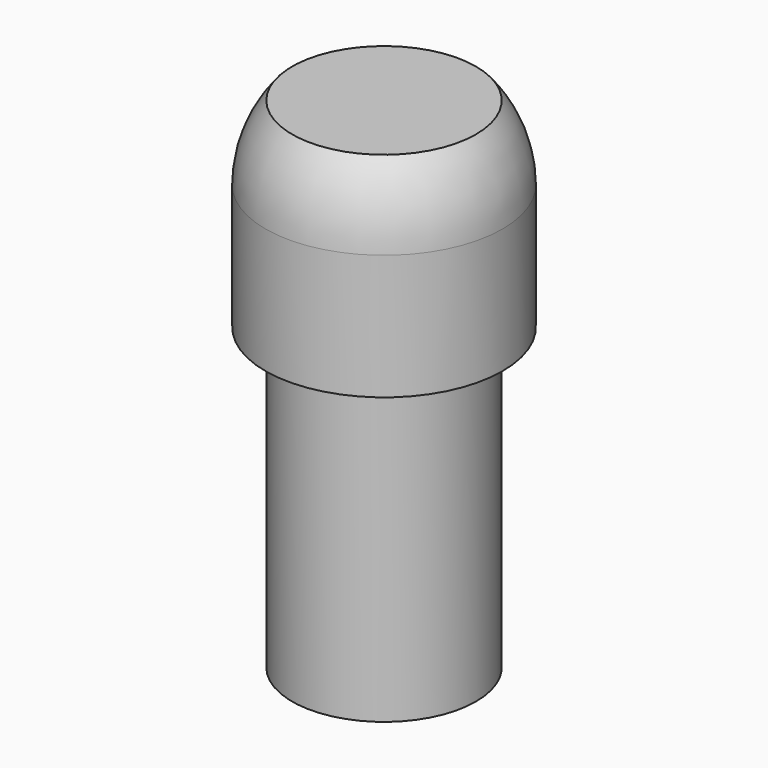
from build123d import *

# Parameters (mm, degrees)
F0_R     = 23.38500022
F1_DEPTH = 76.2
F2_R     = 30.1625
F2_R_2   = 23.38500022
F3_DEPTH = 50.8
F4_DEPTH = 50.8


# Not quite as in the source:
# - a fillet or chamfer that OpenCascade refuses, or shapes differently, is made with other operations: its cross-section is extruded or revolved along the edge and cut away or added


with BuildPart() as f1:
    # F0 (on Top) → F1 (new body)
    with BuildSketch(Plane.XY):
        Circle(F0_R)
    extrude(amount=F1_DEPTH)


with BuildPart() as f3:
    # F2 (on face) → F3 (new body)
    with BuildSketch(Plane.XY.offset(76.2)):
        Circle(F2_R)
        Circle(F2_R_2, mode=Mode.SUBTRACT)
    extrude(amount=F3_DEPTH)

    # F5: fillet of radius 29.972 on 1 edges, made by hand

    # F5_s1 → F5_t2 (revolve, cut)
    with BuildSketch(Plane.XZ):
        with BuildLine():
            ThreePointArc((30.1625, 108.0174832136), (28.4173165456, 118.0955590073), (23.38500022, 127))
            Line((23.38500022, 127), (30.1625, 127))
            Line((30.1625, 127), (30.1625, 108.0174832136))
        make_face()
    revolve(axis=Axis((0, 0, 127), (0, 0, 1)), mode=Mode.SUBTRACT)


with BuildPart() as f4:
    # F4 (new): a face of the model
    f4_faces = [f1.part.faces().sort_by_distance(p)[0] for p in [
        (0, 0, 76.2),
    ]]
    extrude(f4_faces, amount=F4_DEPTH)


solid = Compound([f1.part, f3.part, f4.part])
